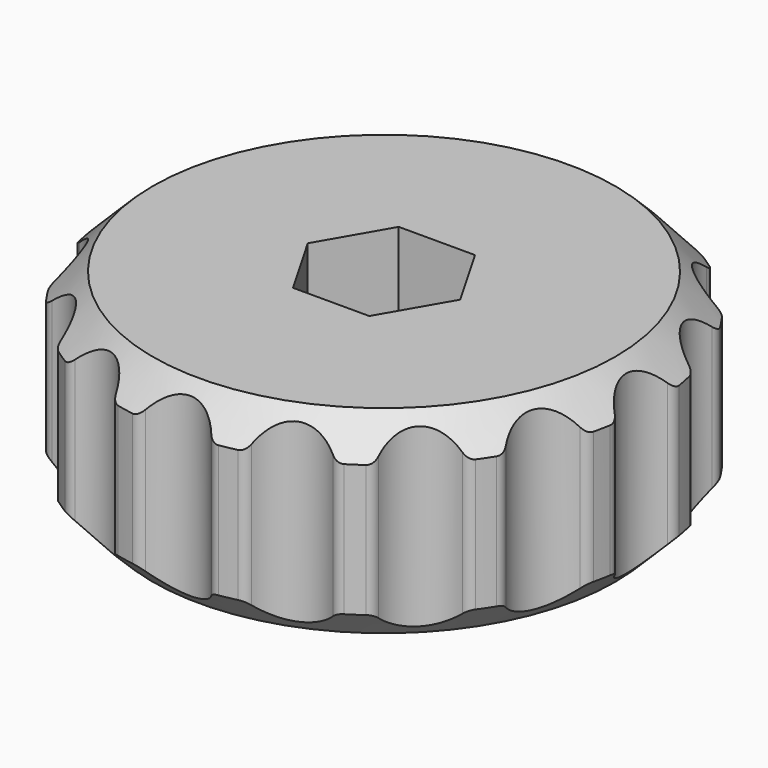
from build123d import *

# Parameters (mm, degrees)
F0_R        = 12
F0_R_2      = 1.65
F1_DEPTH    = 9
F2_SIZE     = 1.5
F4_DEPTH    = 7
F5_R        = 2
F6_DEPTH    = 9.001
F7_T1_DEPTH = 7.4980807946


# Not quite as in the source:
# - a fillet or chamfer that OpenCascade refuses, or shapes differently, is made with other operations: its cross-section is extruded or revolved along the edge and cut away or added


with BuildPart() as f1:
    # F0 (on Top) → F1 (new body)
    with BuildSketch(Plane.XY):
        Circle(F0_R)
        Circle(F0_R_2, mode=Mode.SUBTRACT)
    extrude(amount=F1_DEPTH)

    # F2
    f2_edges = [f1.edges().sort_by_distance(p)[0] for p in [
        (-12, 0, 9),
        (-12, 0, 0),
    ]]
    chamfer(f2_edges, length=F2_SIZE)

    # F3 (on face) → F4 (cut)
    with BuildSketch(Plane.XY.offset(9)):
        Polygon((-1.7320508076, -3), (1.7320508076, -3), (3.4641016151, 0), (1.7320508076, 3), (-1.7320508076, 3), (-3.4641016151, 0), align=None)
    extrude(amount=-F4_DEPTH, mode=Mode.SUBTRACT)

    # F5 (on face) → F6 (cut, through all)
    with BuildSketch(Plane.XY.offset(9)):
        with Locations((13, 0)):
            Circle(F5_R)
        with Locations((12.0104339226, 4.9748846207)):
            Circle(F5_R)
        with Locations((9.1923881554, 9.1923881554)):
            Circle(F5_R)
        with Locations((4.9748846207, 12.0104339226)):
            Circle(F5_R)
        with Locations((0, 13)):
            Circle(F5_R)
        with Locations((-4.9748846207, 12.0104339226)):
            Circle(F5_R)
        with Locations((-9.1923881554, 9.1923881554)):
            Circle(F5_R)
        with Locations((-12.0104339226, 4.9748846207)):
            Circle(F5_R)
        with Locations((-13, 0)):
            Circle(F5_R)
        with Locations((-12.0104339226, -4.9748846207)):
            Circle(F5_R)
        with Locations((-9.1923881554, -9.1923881554)):
            Circle(F5_R)
        with Locations((-4.9748846207, -12.0104339226)):
            Circle(F5_R)
        with Locations((0, -13)):
            Circle(F5_R)
        with Locations((4.9748846207, -12.0104339226)):
            Circle(F5_R)
        with Locations((9.1923881554, -9.1923881554)):
            Circle(F5_R)
        with Locations((12.0104339226, -4.9748846207)):
            Circle(F5_R)
    extrude(amount=-F6_DEPTH, mode=Mode.SUBTRACT)

    # F7: fillet of radius 0.5 on 32 edges, made by hand

    # F7_s2 → F7_t1 (cut)
    with BuildSketch(Plane.XY.offset(0.7509596027)):
        with BuildLine():
            ThreePointArc((-1.9562901844, 11.8394648829), (-1.7070514239, 11.8171822576), (-1.4998224747, 11.6769230769))
            ThreePointArc((-1.4998224747, 11.6769230769), (-1.5833680774, 11.7781384974), (-1.6600955273, 11.8846153846))
            ThreePointArc((-1.6600955273, 11.8846153846), (-1.8083337761, 11.8629645938), (-1.9562901844, 11.8394648829))
        make_face()
        with BuildLine():
            ThreePointArc((1.4998224747, 11.6769230769), (1.7070514239, 11.8171822576), (1.9562901844, 11.8394648829))
            ThreePointArc((1.9562901844, 11.8394648829), (1.8083337761, 11.8629645938), (1.6600955273, 11.8846153846))
            ThreePointArc((1.6600955273, 11.8846153846), (1.5833680774, 11.7781384974), (1.4998224747, 11.6769230769))
        make_face()
        with BuildLine():
            ThreePointArc((2.7233905978, 11.6868791237), (2.9451299957, 11.5709131178), (3.0829097158, 11.362027446))
            ThreePointArc((3.0829097158, 11.362027446), (3.0444571079, 11.4875098194), (3.014317128, 11.6152439601))
            ThreePointArc((3.014317128, 11.6152439601), (2.8690774451, 11.6519695594), (2.7233905978, 11.6868791237))
        make_face()
        with BuildLine():
            ThreePointArc((5.8542202893, 10.2141130209), (6.0993497387, 10.2643925216), (6.3381435198, 10.1895994388))
            ThreePointArc((6.3381435198, 10.1895994388), (6.2104425725, 10.2679308068), (6.0817736874, 10.3446618512))
            ThreePointArc((6.0817736874, 10.3446618512), (5.9701398262, 10.2756523583), (5.8542202893, 10.2141130209))
        make_face()
        with BuildLine():
            ThreePointArc((6.988459849, 9.7550719597), (7.1489420712, 9.5630773465), (7.1962968486, 9.3173661335))
            ThreePointArc((7.1962968486, 9.3173661335), (7.2087912966, 9.4480119059), (7.2298273255, 9.577556935))
            ThreePointArc((7.2298273255, 9.577556935), (7.1096976335, 9.667067785), (6.988459849, 9.7550719597))
        make_face()
        with BuildLine():
            ThreePointArc((9.3173661335, 7.1962968486), (9.5630773465, 7.1489420712), (9.7550719597, 6.988459849))
            ThreePointArc((9.7550719597, 6.988459849), (9.667067785, 7.1096976335), (9.577556935, 7.2298273255))
            ThreePointArc((9.577556935, 7.2298273255), (9.4480119059, 7.2087912966), (9.3173661335, 7.1962968486))
        make_face()
        with BuildLine():
            ThreePointArc((11.6868791237, 2.7233905978), (11.5709131178, 2.9451299957), (11.362027446, 3.0829097158))
            ThreePointArc((11.362027446, 3.0829097158), (11.4875098194, 3.0444571079), (11.6152439601, 3.014317128))
            ThreePointArc((11.6152439601, 3.014317128), (11.6519695594, 2.8690774451), (11.6868791237, 2.7233905978))
        make_face()
        with BuildLine():
            ThreePointArc((10.1895994388, 6.3381435198), (10.2643925216, 6.0993497387), (10.2141130209, 5.8542202893))
            ThreePointArc((10.2141130209, 5.8542202893), (10.2756523583, 5.9701398262), (10.3446618512, 6.0817736874))
            ThreePointArc((10.3446618512, 6.0817736874), (10.2679308068, 6.2104425725), (10.1895994388, 6.3381435198))
        make_face()
        with BuildLine():
            ThreePointArc((11.8394648829, 1.9562901844), (11.8171822576, 1.7070514239), (11.6769230769, 1.4998224747))
            ThreePointArc((11.6769230769, 1.4998224747), (11.7781384974, 1.5833680774), (11.8846153846, 1.6600955273))
            ThreePointArc((11.8846153846, 1.6600955273), (11.8629645938, 1.8083337761), (11.8394648829, 1.9562901844))
        make_face()
        with BuildLine():
            ThreePointArc((11.6769230769, -1.4998224747), (11.8171822576, -1.7070514239), (11.8394648829, -1.9562901844))
            ThreePointArc((11.8394648829, -1.9562901844), (11.8629645938, -1.8083337761), (11.8846153846, -1.6600955273))
            ThreePointArc((11.8846153846, -1.6600955273), (11.7781384974, -1.5833680774), (11.6769230769, -1.4998224747))
        make_face()
        with BuildLine():
            ThreePointArc((11.6868791237, -2.7233905978), (11.5709131178, -2.9451299957), (11.362027446, -3.0829097158))
            ThreePointArc((11.362027446, -3.0829097158), (11.4875098194, -3.0444571079), (11.6152439601, -3.014317128))
            ThreePointArc((11.6152439601, -3.014317128), (11.6519695594, -2.8690774451), (11.6868791237, -2.7233905978))
        make_face()
        with BuildLine():
            ThreePointArc((10.2141130209, -5.8542202893), (10.2643925216, -6.0993497387), (10.1895994388, -6.3381435198))
            ThreePointArc((10.1895994388, -6.3381435198), (10.2679308068, -6.2104425725), (10.3446618512, -6.0817736874))
            ThreePointArc((10.3446618512, -6.0817736874), (10.2756523583, -5.9701398262), (10.2141130209, -5.8542202893))
        make_face()
        with BuildLine():
            ThreePointArc((9.7550719597, -6.988459849), (9.5630773465, -7.1489420712), (9.3173661335, -7.1962968486))
            ThreePointArc((9.3173661335, -7.1962968486), (9.4480119059, -7.2087912966), (9.577556935, -7.2298273255))
            ThreePointArc((9.577556935, -7.2298273255), (9.667067785, -7.1096976335), (9.7550719597, -6.988459849))
        make_face()
        with BuildLine():
            ThreePointArc((7.1962968486, -9.3173661335), (7.1489420712, -9.5630773465), (6.988459849, -9.7550719597))
            ThreePointArc((6.988459849, -9.7550719597), (7.1096976335, -9.667067785), (7.2298273255, -9.577556935))
            ThreePointArc((7.2298273255, -9.577556935), (7.2087912966, -9.4480119059), (7.1962968486, -9.3173661335))
        make_face()
        with BuildLine():
            ThreePointArc((6.3381435198, -10.1895994388), (6.0993497387, -10.2643925216), (5.8542202893, -10.2141130209))
            ThreePointArc((5.8542202893, -10.2141130209), (5.9701398262, -10.2756523583), (6.0817736874, -10.3446618512))
            ThreePointArc((6.0817736874, -10.3446618512), (6.2104425725, -10.2679308068), (6.3381435198, -10.1895994388))
        make_face()
        with BuildLine():
            ThreePointArc((3.0829097158, -11.362027446), (2.9451299957, -11.5709131178), (2.7233905978, -11.6868791237))
            ThreePointArc((2.7233905978, -11.6868791237), (2.8690774451, -11.6519695594), (3.014317128, -11.6152439601))
            ThreePointArc((3.014317128, -11.6152439601), (3.0444571079, -11.4875098194), (3.0829097158, -11.362027446))
        make_face()
        with BuildLine():
            ThreePointArc((1.9562901844, -11.8394648829), (1.7070514239, -11.8171822576), (1.4998224747, -11.6769230769))
            ThreePointArc((1.4998224747, -11.6769230769), (1.5833680774, -11.7781384974), (1.6600955273, -11.8846153846))
            ThreePointArc((1.6600955273, -11.8846153846), (1.8083337761, -11.8629645938), (1.9562901844, -11.8394648829))
        make_face()
        with BuildLine():
            ThreePointArc((-1.4998224747, -11.6769230769), (-1.7070514239, -11.8171822576), (-1.9562901844, -11.8394648829))
            ThreePointArc((-1.9562901844, -11.8394648829), (-1.8083337761, -11.8629645938), (-1.6600955273, -11.8846153846))
            ThreePointArc((-1.6600955273, -11.8846153846), (-1.5833680774, -11.7781384974), (-1.4998224747, -11.6769230769))
        make_face()
        with BuildLine():
            ThreePointArc((-2.7233905978, -11.6868791237), (-2.9451299957, -11.5709131178), (-3.0829097158, -11.362027446))
            ThreePointArc((-3.0829097158, -11.362027446), (-3.0444571079, -11.4875098194), (-3.014317128, -11.6152439601))
            ThreePointArc((-3.014317128, -11.6152439601), (-2.8690774451, -11.6519695594), (-2.7233905978, -11.6868791237))
        make_face()
        with BuildLine():
            ThreePointArc((-5.8542202893, -10.2141130209), (-6.0993497387, -10.2643925216), (-6.3381435198, -10.1895994388))
            ThreePointArc((-6.3381435198, -10.1895994388), (-6.2104425725, -10.2679308068), (-6.0817736874, -10.3446618512))
            ThreePointArc((-6.0817736874, -10.3446618512), (-5.9701398262, -10.2756523583), (-5.8542202893, -10.2141130209))
        make_face()
        with BuildLine():
            ThreePointArc((-6.988459849, -9.7550719597), (-7.1489420712, -9.5630773465), (-7.1962968486, -9.3173661335))
            ThreePointArc((-7.1962968486, -9.3173661335), (-7.2087912966, -9.4480119059), (-7.2298273255, -9.577556935))
            ThreePointArc((-7.2298273255, -9.577556935), (-7.1096976335, -9.667067785), (-6.988459849, -9.7550719597))
        make_face()
        with BuildLine():
            ThreePointArc((-9.3173661335, -7.1962968486), (-9.5630773465, -7.1489420712), (-9.7550719597, -6.988459849))
            ThreePointArc((-9.7550719597, -6.988459849), (-9.667067785, -7.1096976335), (-9.577556935, -7.2298273255))
            ThreePointArc((-9.577556935, -7.2298273255), (-9.4480119059, -7.2087912966), (-9.3173661335, -7.1962968486))
        make_face()
        with BuildLine():
            ThreePointArc((-10.1895994388, -6.3381435198), (-10.2643925216, -6.0993497387), (-10.2141130209, -5.8542202893))
            ThreePointArc((-10.2141130209, -5.8542202893), (-10.2756523583, -5.9701398262), (-10.3446618512, -6.0817736874))
            ThreePointArc((-10.3446618512, -6.0817736874), (-10.2679308068, -6.2104425725), (-10.1895994388, -6.3381435198))
        make_face()
        with BuildLine():
            ThreePointArc((-11.362027446, -3.0829097158), (-11.5709131178, -2.9451299957), (-11.6868791237, -2.7233905978))
            ThreePointArc((-11.6868791237, -2.7233905978), (-11.6519695594, -2.8690774451), (-11.6152439601, -3.014317128))
            ThreePointArc((-11.6152439601, -3.014317128), (-11.4875098194, -3.0444571079), (-11.362027446, -3.0829097158))
        make_face()
        with BuildLine():
            ThreePointArc((-11.8394648829, -1.9562901844), (-11.8171822576, -1.7070514239), (-11.6769230769, -1.4998224747))
            ThreePointArc((-11.6769230769, -1.4998224747), (-11.7781384974, -1.5833680774), (-11.8846153846, -1.6600955273))
            ThreePointArc((-11.8846153846, -1.6600955273), (-11.8629645938, -1.8083337761), (-11.8394648829, -1.9562901844))
        make_face()
        with BuildLine():
            ThreePointArc((-11.6769230769, 1.4998224747), (-11.8171822576, 1.7070514239), (-11.8394648829, 1.9562901844))
            ThreePointArc((-11.8394648829, 1.9562901844), (-11.8629645938, 1.8083337761), (-11.8846153846, 1.6600955273))
            ThreePointArc((-11.8846153846, 1.6600955273), (-11.7781384974, 1.5833680774), (-11.6769230769, 1.4998224747))
        make_face()
        with BuildLine():
            ThreePointArc((-11.6868791237, 2.7233905978), (-11.5709131178, 2.9451299957), (-11.362027446, 3.0829097158))
            ThreePointArc((-11.362027446, 3.0829097158), (-11.4875098194, 3.0444571079), (-11.6152439601, 3.014317128))
            ThreePointArc((-11.6152439601, 3.014317128), (-11.6519695594, 2.8690774451), (-11.6868791237, 2.7233905978))
        make_face()
        with BuildLine():
            ThreePointArc((-10.2141130209, 5.8542202893), (-10.2643925216, 6.0993497387), (-10.1895994388, 6.3381435198))
            ThreePointArc((-10.1895994388, 6.3381435198), (-10.2679308068, 6.2104425725), (-10.3446618512, 6.0817736874))
            ThreePointArc((-10.3446618512, 6.0817736874), (-10.2756523583, 5.9701398262), (-10.2141130209, 5.8542202893))
        make_face()
        with BuildLine():
            ThreePointArc((-9.7550719597, 6.988459849), (-9.5630773465, 7.1489420712), (-9.3173661335, 7.1962968486))
            ThreePointArc((-9.3173661335, 7.1962968486), (-9.4480119059, 7.2087912966), (-9.577556935, 7.2298273255))
            ThreePointArc((-9.577556935, 7.2298273255), (-9.667067785, 7.1096976335), (-9.7550719597, 6.988459849))
        make_face()
        with BuildLine():
            ThreePointArc((-7.1962968486, 9.3173661335), (-7.1489420712, 9.5630773465), (-6.988459849, 9.7550719597))
            ThreePointArc((-6.988459849, 9.7550719597), (-7.1096976335, 9.667067785), (-7.2298273255, 9.577556935))
            ThreePointArc((-7.2298273255, 9.577556935), (-7.2087912966, 9.4480119059), (-7.1962968486, 9.3173661335))
        make_face()
        with BuildLine():
            ThreePointArc((-6.3381435198, 10.1895994388), (-6.0993497387, 10.2643925216), (-5.8542202893, 10.2141130209))
            ThreePointArc((-5.8542202893, 10.2141130209), (-5.9701398262, 10.2756523583), (-6.0817736874, 10.3446618512))
            ThreePointArc((-6.0817736874, 10.3446618512), (-6.2104425725, 10.2679308068), (-6.3381435198, 10.1895994388))
        make_face()
        with BuildLine():
            ThreePointArc((-3.0829097158, 11.362027446), (-2.9451299957, 11.5709131178), (-2.7233905978, 11.6868791237))
            ThreePointArc((-2.7233905978, 11.6868791237), (-2.8690774451, 11.6519695594), (-3.014317128, 11.6152439601))
            ThreePointArc((-3.014317128, 11.6152439601), (-3.0444571079, 11.4875098194), (-3.0829097158, 11.362027446))
        make_face()
    extrude(amount=F7_T1_DEPTH, mode=Mode.SUBTRACT)


solid = f1.part
